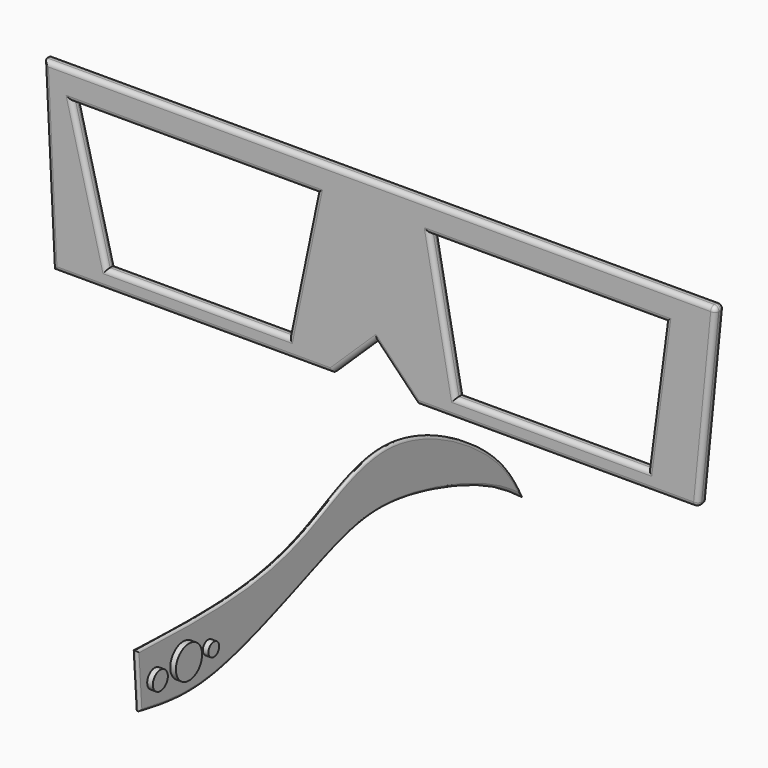
from build123d import *

# Parameters (mm, degrees)
F1_DEPTH = 2.54
F2_R     = 1.016
F4_DEPTH = 1.016
F5_R     = 0.5079
F6_R     = 3.6731561764
F6_R_2   = 2.1012773658
F6_R_3   = 1.5151331211
F7_DEPTH = 1.27


# Not quite as in the source:
# - a fillet or chamfer is up to 0.001 mm smaller than in the source, because OpenCascade refuses the exact size


with BuildPart() as f1:
    # F0 (on Front) → F1 (new body)
    with BuildSketch(Plane.XZ):
        Polygon((76.2685239315, 31.3708260655), (-74.541695416, 31.3708260655), (-72.527050972, -9.497590363), (-9.7943909623, -9.497590363), (0, 0), (9.2097837478, -9.497590363), (72.2392424941, -9.497590363), align=None)
        Polygon((-60.4392103851, -5.4683093913), (-68.2099610567, 25.0390991569), (-13.2390642539, 25.0390991569), (-19.5707920939, -5.4683093913), align=None, mode=Mode.SUBTRACT)
        Polygon((17.8439579904, -5.4683093913), (12.0878405869, 25.0390991569), (65.0441050529, 25.0390991569), (61.0148236156, -5.4683093913), align=None, mode=Mode.SUBTRACT)
    extrude(amount=F1_DEPTH)

    # F2
    f2_edges = [f1.edges().sort_by_distance(p)[0] for p in [
        (-41.160721, -2.54, -9.49759),
        (-41.160721, 0, -9.49759),
        (40.724513, -2.54, -9.49759),
        (-4.897195, -2.54, -4.748795),
        (-4.897195, 0, -4.748795),
        (40.724513, 0, -9.49759),
        (0.863414, -2.54, 31.370826),
        (0.863414, 0, 31.370826),
        (74.253883, -2.54, 10.936618),
        (72.239242, -1.27, -9.49759),
        (76.268524, -1.27, 31.370826),
        (74.253883, 0, 10.936618),
        (-73.534373, -2.54, 10.936618),
        (-73.534373, 0, 10.936618),
        (63.029464, 0, 9.785395),
        (63.029464, -2.54, 9.785395),
        (38.565973, 0, 25.039099),
        (38.565973, -2.54, 25.039099),
        (-40.724513, -2.54, 25.039099),
        (-40.724513, 0, 25.039099),
        (-16.404928, 0, 9.785395),
        (-16.404928, -2.54, 9.785395),
        (14.965899, -2.54, 9.785395),
        (14.965899, 0, 9.785395),
        (-40.005001, -2.54, -5.468309),
        (-40.005001, 0, -5.468309),
        (-64.324586, -2.54, 9.785395),
        (-64.324586, 0, 9.785395),
        (39.429391, 0, -5.468309),
        (39.429391, -2.54, -5.468309),
        (4.604892, -2.54, -4.748795),
        (4.604892, 0, -4.748795),
    ]]
    fillet(f2_edges, radius=F2_R)


with BuildPart() as f4:
    # F3 (on Right) → F4 (new body)
    with BuildSketch(Plane.YZ):
        with BuildLine():
            add(Edge.make_bspline(
                [(-70.8002150059, -33.0976620317), (-70.5124090115, -37.2228771448), (-70.2246030172, -41.348092258), (-69.9367970228, -45.4733073711)],
                knots=[0, 0, 0, 0, 12.4057280392, 12.4057280392, 12.4057280392, 12.4057280392], degree=3))
            add(Edge.make_bspline(
                [(-69.9367970228, -45.4733073711), (-63.8069137805, -46.6217839294), (-49.8536971797, -49.236016786), (-18.8753087346, -35.9150239322), (-0.9804728035, -30.4416104122), (27.4700571362, -39.2796131228), (34.7758176291, -44.729198934), (37.7025529742, -46.9123385847)],
                knots=[0, 0, 0, 0, 0.1904106072, 0.4334243151, 0.6226378654, 0.8488262655, 1, 1, 1, 1], degree=3))
            add(Edge.make_bspline(
                [(-70.8002150059, -33.0976620317), (-61.2142736716, -33.4184012283), (-43.2817896772, -34.0184101695), (-22.3538595554, -29.876760887), (-0.4687688132, -15.568770675), (30.580842513, -33.6877378685), (35.6582136421, -43.1161197489), (37.7025529742, -46.9123385847)],
                knots=[0, 0, 0, 0, 0.2170842724, 0.4061009872, 0.6077837092, 0.8420790662, 1, 1, 1, 1], degree=3))
        make_face()
    extrude(amount=F4_DEPTH)

    # F5 (radius 0.508 in the source; OpenCascade refuses exactly that, so slightly less here)
    f5_edges = [f4.edges().sort_by_distance(p)[0] for p in [
        (1.016, -12.322711, -23.785699),
        (1.016, -15.465077, -35.16226),
        (1.016, -70.368506, -39.285485),
        (0, -15.465077, -35.16226),
        (0, -70.368506, -39.285485),
        (0, -12.322711, -23.785699),
    ]]
    fillet(f5_edges, radius=F5_R)

    # F6 (on face) → F7 (join)
    with BuildSketch(Plane.YZ.offset(1.016)):
        with Locations((-57.8121580184, -40.0984920561)):
            Circle(F6_R)
        with Locations((-65.8440813422, -40.4783003032)):
            Circle(F6_R_2)
        with Locations((-50.8401691914, -40.4247641563)):
            Circle(F6_R_3)
    extrude(amount=F7_DEPTH)


solid = Compound([f1.part, f4.part])
